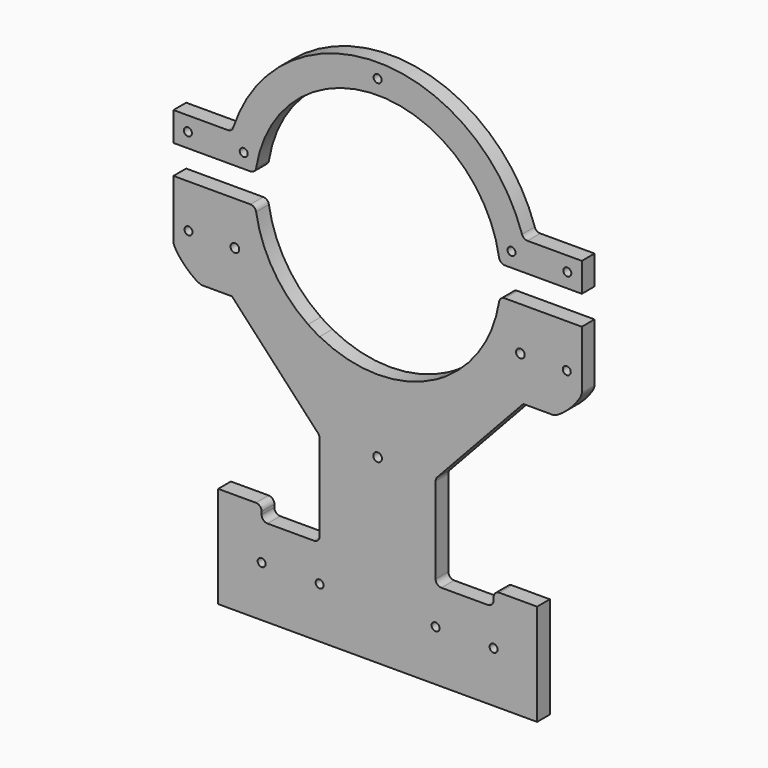
from build123d import *

# Parameters (mm, degrees)
F0_W        = 3.1917378622
F0_H        = 20
F0_R        = 1.5
F0_W_2      = 4.8082621378
F0_R_2      = 1.38
F0_H_2      = 10
F1_DEPTH    = 5.5
F0_W_3      = 10
F2_R        = 2
F2_2_R      = 2
F3_T1_DEPTH = 55.5


# Not quite as in the source:
# - a fillet or chamfer that OpenCascade refuses, or shapes differently, is made with other operations: its cross-section is extruded or revolved along the edge and cut away or added


with BuildPart() as f1:
    # F0 (on Front) → F1 (new body)
    with BuildSketch(Plane.XZ):
        with Locations((-58.8291310689, 115)):
            Rectangle(F0_W, F0_H)
        with BuildLine():
            Line((-52.425, 95), (-50.2332621378, 95))
            Line((-50.2332621378, 95), (-23.9766683465, 95))
            ThreePointArc((-23.9766683465, 95), (-36.2973941829, 108.0368535831), (-42.1293321215, 125))
            Line((-42.1293321215, 125), (-52.425, 125))
            Line((-52.425, 125), (-52.425, 105))
            Line((-52.425, 105), (-52.425, 95))
        make_face()
        with Locations((-49.2332621378, 110)):
            Circle(F0_R, mode=Mode.SUBTRACT)
        with Locations((58.8291310689, 115)):
            Rectangle(F0_W, F0_H)
        with Locations((54.8291310689, 115)):
            Rectangle(F0_W_2, F0_H)
        with BuildLine():
            Line((-20, 62.5), (-20, 30))
            Line((-20, 30), (20, 30))
            Line((20, 30), (20, 62.5))
            Line((20, 62.5), (20, 92.5850213818))
            ThreePointArc((20, 92.5850213818), (0, 87.575), (-20, 92.5850213818))
            Line((-20, 92.5850213818), (-20, 62.5))
        make_face()
        with Locations((0, 62.5)):
            Circle(F0_R, mode=Mode.SUBTRACT)
        Polygon((-30, 30), (-30, 0), (30, 0), (30, 30), (20, 30), (-20, 30), align=None)
        with Locations((-20, 17.5)):
            Circle(F0_R_2, mode=Mode.SUBTRACT)
        with Locations((20, 17.5)):
            Circle(F0_R_2, mode=Mode.SUBTRACT)
        Polygon((-70.425, 95), (-60.425, 95), (-60.425, 105), (-60.425, 125), (-70.425, 125), align=None)
        with Locations((-65.2332621378, 110)):
            Circle(F0_R_2, mode=Mode.SUBTRACT)
        with Locations((-58.8291310689, 100)):
            Rectangle(F0_W, F0_H_2)
        with Locations((-54.8291310689, 100)):
            Rectangle(F0_W_2, F0_H_2)
        with Locations((54.8291310689, 100)):
            Rectangle(F0_W_2, F0_H_2)
        with Locations((58.8291310689, 100)):
            Rectangle(F0_W, F0_H_2)
        Polygon((60.425, 105), (60.425, 95), (70.425, 95), (70.425, 125), (60.425, 125), align=None)
        with Locations((65.2332621378, 110)):
            Circle(F0_R_2, mode=Mode.SUBTRACT)
        with BuildLine():
            Line((-40, 16.12), (-40, 0))
            Line((-40, 0), (-30, 0))
            Line((-30, 0), (-30, 30))
            Line((-30, 30), (-40, 30))
            Line((-40, 30), (-40, 18.88))
            ThreePointArc((-40, 18.88), (-39.024192642, 18.475807358), (-38.62, 17.5))
            ThreePointArc((-38.62, 17.5), (-39.024192642, 16.524192642), (-40, 16.12))
        make_face()
        with BuildLine():
            Line((-55, 0), (-40, 0))
            Line((-40, 0), (-40, 16.12))
            ThreePointArc((-40, 16.12), (-41.38, 17.5), (-40, 18.88))
            Line((-40, 18.88), (-40, 30))
            Line((-40, 30), (-40, 35))
            Line((-40, 35), (-55, 35))
            Line((-55, 35), (-55, 0))
        make_face()
        with BuildLine():
            Line((40, 16.12), (40, 0))
            Line((40, 0), (55, 0))
            Line((55, 0), (55, 35))
            Line((55, 35), (40, 35))
            Line((40, 35), (40, 30))
            Line((40, 30), (40, 18.88))
            ThreePointArc((40, 18.88), (40.975807358, 18.475807358), (41.38, 17.5))
            ThreePointArc((41.38, 17.5), (40.975807358, 16.524192642), (40, 16.12))
        make_face()
        with BuildLine():
            Line((30, 30), (30, 0))
            Line((30, 0), (40, 0))
            Line((40, 0), (40, 16.12))
            ThreePointArc((40, 16.12), (38.62, 17.5), (40, 18.88))
            Line((40, 18.88), (40, 30))
            Line((40, 30), (30, 30))
        make_face()
        with BuildLine():
            Line((20, 92.5850213818), (20, 62.5))
            Line((20, 62.5), (50.2332621378, 95))
            Line((50.2332621378, 95), (23.9766683465, 95))
            ThreePointArc((23.9766683465, 95), (22.0214638511, 93.7379571059), (20, 92.5850213818))
        make_face()
        with BuildLine():
            Line((-50.2332621378, 95), (-20, 62.5))
            Line((-20, 62.5), (-20, 92.5850213818))
            ThreePointArc((-20, 92.5850213818), (-22.0214638511, 93.7379571059), (-23.9766683465, 95))
            Line((-23.9766683465, 95), (-50.2332621378, 95))
        make_face()
        with BuildLine():
            Line((23.9766683465, 95), (50.2332621378, 95))
            Line((50.2332621378, 95), (52.425, 95))
            Line((52.425, 95), (52.425, 105))
            Line((52.425, 105), (52.425, 125))
            Line((52.425, 125), (42.1293321215, 125))
            ThreePointArc((42.1293321215, 125), (36.2973941829, 108.0368535831), (23.9766683465, 95))
        make_face()
        with Locations((49.2332621378, 110)):
            Circle(F0_R, mode=Mode.SUBTRACT)
        with Locations((-54.8291310689, 115)):
            Rectangle(F0_W_2, F0_H)
    extrude(amount=F1_DEPTH)

    # F2
    f2_edges = [f1.edges().sort_by_distance(p)[0] for p in [
        (-40, -2.75, 30),
        (-40, -2.75, 35),
        (-20, -2.75, 30),
        (20, -2.75, 30),
        (40, -2.75, 30),
        (40, -2.75, 35),
        (-42.129332, -2.75, 125),
        (42.129332, -2.75, 125),
        (-20, -2.75, 62.5),
        (20, -2.75, 62.5),
    ]]
    fillet(f2_edges, radius=F2_R)

    # F3: fillet of radius 10 on 2 edges, made by hand

    # F3_s2 → F3_t1 (cut)
    with BuildSketch(Plane.XZ.offset(-25)):
        with BuildLine():
            add(Edge.make_bspline(
                [(-60.425, 95), (-70.425, 95), (-70.425, 105)],
                knots=[0, 0, 0, 1, 1, 1], degree=2, weights=[1, 0.25, 1]))
            Line((-70.425, 105), (-70.425, 95))
            Line((-70.425, 95), (-60.425, 95))
        make_face()
        with BuildLine():
            add(Edge.make_bspline(
                [(70.425, 105), (70.425, 95), (60.425, 95)],
                knots=[0, 0, 0, 1, 1, 1], degree=2, weights=[1, 0.25, 1]))
            Line((60.425, 95), (70.425, 95))
            Line((70.425, 95), (70.425, 105))
        make_face()
    extrude(amount=F3_T1_DEPTH, mode=Mode.SUBTRACT)


with BuildPart() as f1b:
    # F0 (on Front) → F1, piece 2 (new body)
    with BuildSketch(Plane.XZ):
        with BuildLine():
            Line((42.1293321215, 135), (57.2332621378, 135))
            Line((57.2332621378, 135), (57.2332621378, 145))
            Line((57.2332621378, 145), (50.2332621378, 145))
            ThreePointArc((50.2332621378, 145), (0, 182.425), (-50.2332621378, 145))
            Line((-50.2332621378, 145), (-57.2332621378, 145))
            Line((-57.2332621378, 145), (-57.2332621378, 135))
            Line((-57.2332621378, 135), (-42.1293321215, 135))
            ThreePointArc((-42.1293321215, 135), (0, 172.425), (42.1293321215, 135))
        make_face()
        with Locations((-46.1812971296, 140)):
            Circle(F0_R_2, mode=Mode.SUBTRACT)
        with Locations((0, 177.425)):
            Circle(F0_R_2, mode=Mode.SUBTRACT)
        with Locations((46.1812971296, 140)):
            Circle(F0_R_2, mode=Mode.SUBTRACT)
        with Locations((58.8291310689, 140)):
            Rectangle(F0_W, F0_H_2)
        with Locations((-58.8291310689, 140)):
            Rectangle(F0_W, F0_H_2)
        with Locations((-65.425, 140)):
            Rectangle(F0_W_3, F0_H_2)
        with Locations((-65.425, 140)):
            Circle(F0_R_2, mode=Mode.SUBTRACT)
        with Locations((65.425, 140)):
            Rectangle(F0_W_3, F0_H_2)
        with Locations((65.425, 140)):
            Circle(F0_R_2, mode=Mode.SUBTRACT)
    extrude(amount=F1_DEPTH)

    # F2#2
    f2_2_edges = [f1b.edges().sort_by_distance(p)[0] for p in [
        (-50.233262, -2.75, 145),
        (50.233262, -2.75, 145),
        (-42.129332, -2.75, 135),
        (42.129332, -2.75, 135),
    ]]
    fillet(f2_2_edges, radius=F2_2_R)


solid = Compound([f1.part, f1b.part])
